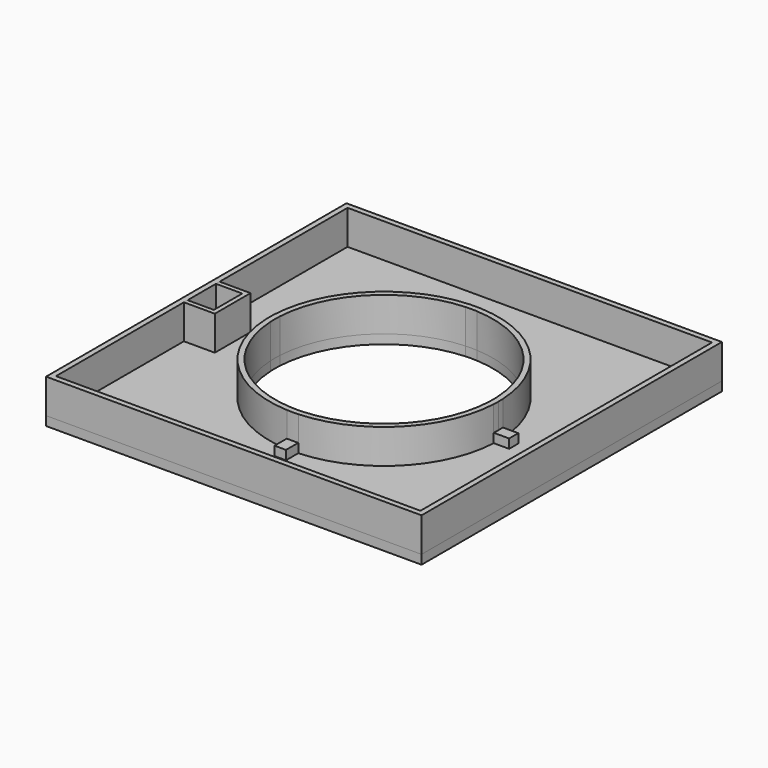
from build123d import *

# Parameters (mm, degrees)
F1_DEPTH = 7.5
F0_W     = 82
F0_H     = 82
F0_R     = 32.8
F0_W_2   = 6.75
F0_H_2   = 9.75
F2_DEPTH = 2
F3_DEPTH = 2
F4_DEPTH = 7.5
F5_T     = -1


# Not quite as in the source:
# - a feature names something its author has since deleted; it is built from what else it names


with BuildPart() as f1:
    # F0 (on Top) → F1 (new body)
    with BuildSketch(Plane.XY):
        with BuildLine():
            ThreePointArc((-24.9687304443, -1.25), (-17.6776695297, -17.6776695297), (-1.25, -24.9687304443))
            Line((-1.25, -24.9687304443), (-1.25, -23.7671517015))
            ThreePointArc((-1.25, -23.7671517015), (-16.8291413922, -16.8291413922), (-23.7671517015, -1.25))
            Line((-23.7671517015, -1.25), (-24.9687304443, -1.25))
        make_face()
        with BuildLine():
            Line((-1.25, 23.7671517015), (-1.25, 24.9687304443))
            ThreePointArc((-1.25, 24.9687304443), (-17.6776695297, 17.6776695297), (-24.9687304443, 1.25))
            Line((-24.9687304443, 1.25), (-23.7671517015, 1.25))
            ThreePointArc((-23.7671517015, 1.25), (-16.8291413922, 16.8291413922), (-1.25, 23.7671517015))
        make_face()
        with BuildLine():
            Line((23.7671517015, 1.25), (24.9687304443, 1.25))
            ThreePointArc((24.9687304443, 1.25), (17.6776695297, 17.6776695297), (1.25, 24.9687304443))
            Line((1.25, 24.9687304443), (1.25, 23.7671517015))
            ThreePointArc((1.25, 23.7671517015), (16.8291413922, 16.8291413922), (23.7671517015, 1.25))
        make_face()
        with BuildLine():
            ThreePointArc((1.25, -24.9687304443), (17.6776695297, -17.6776695297), (24.9687304443, -1.25))
            Line((24.9687304443, -1.25), (23.7671517015, -1.25))
            ThreePointArc((23.7671517015, -1.25), (16.8291413922, -16.8291413922), (1.25, -23.7671517015))
            Line((1.25, -23.7671517015), (1.25, -24.9687304443))
        make_face()
        with BuildLine():
            Line((1.25, 23.7671517015), (1.25, 24.9687304443))
            ThreePointArc((1.25, 24.9687304443), (0, 25), (-1.25, 24.9687304443))
            Line((-1.25, 24.9687304443), (-1.25, 23.7671517015))
            ThreePointArc((-1.25, 23.7671517015), (0, 23.8), (1.25, 23.7671517015))
        make_face()
        with BuildLine():
            ThreePointArc((-1.25, -24.9687304443), (0, -25), (1.25, -24.9687304443))
            Line((1.25, -24.9687304443), (1.25, -23.7671517015))
            ThreePointArc((1.25, -23.7671517015), (0, -23.8), (-1.25, -23.7671517015))
            Line((-1.25, -23.7671517015), (-1.25, -24.9687304443))
        make_face()
        with BuildLine():
            ThreePointArc((24.9687304443, -1.25), (24.9921813885, -0.6251955264), (25, 0))
            ThreePointArc((25, 0), (24.9921813885, 0.6251955264), (24.9687304443, 1.25))
            Line((24.9687304443, 1.25), (23.7671517015, 1.25))
            ThreePointArc((23.7671517015, 1.25), (23.7917865081, 0.6252157649), (23.8, 0))
            ThreePointArc((23.8, 0), (23.7917865081, -0.6252157649), (23.7671517015, -1.25))
            Line((23.7671517015, -1.25), (24.9687304443, -1.25))
        make_face()
        with BuildLine():
            Line((-23.7671517015, 1.25), (-24.9687304443, 1.25))
            ThreePointArc((-24.9687304443, 1.25), (-25, 0), (-24.9687304443, -1.25))
            Line((-24.9687304443, -1.25), (-23.7671517015, -1.25))
            ThreePointArc((-23.7671517015, -1.25), (-23.8, 0), (-23.7671517015, 1.25))
        make_face()
    extrude(amount=F1_DEPTH)


with BuildPart() as f1b:
    # F0 (on Top) → F1, piece 2 (new body)
    with BuildSketch(Plane.XY):
        Rectangle(F0_W, F0_H)
        Polygon((-39.8, 4.875), (-39.8, 39.8), (39.8, 39.8), (39.8, -39.8), (-39.8, -39.8), (-39.8, -4.875), align=None, mode=Mode.SUBTRACT)
    extrude(amount=F1_DEPTH)


with BuildPart() as f2:
    # F0 (on Top) → F2 (new body)
    with BuildSketch(Plane.XY):
        Rectangle(F0_W, F0_H)
        Polygon((-39.8, 4.875), (-39.8, 39.8), (39.8, 39.8), (39.8, -39.8), (-39.8, -39.8), (-39.8, -4.875), align=None, mode=Mode.SUBTRACT)
        Polygon((39.8, 39.8), (-39.8, 39.8), (-39.8, 4.875), (-33.05, 4.875), (-33.05, -4.875), (-39.8, -4.875), (-39.8, -39.8), (39.8, -39.8), align=None)
        Circle(F0_R, mode=Mode.SUBTRACT)
        Circle(F0_R)
        with BuildLine():
            ThreePointArc((1.25, 24.9687304443), (17.6776695297, 17.6776695297), (24.9687304443, 1.25))
            Line((24.9687304443, 1.25), (28.325, 1.25))
            Line((28.325, 1.25), (28.325, -1.25))
            Line((28.325, -1.25), (24.9687304443, -1.25))
            ThreePointArc((24.9687304443, -1.25), (17.6776695297, -17.6776695297), (1.25, -24.9687304443))
            Line((1.25, -24.9687304443), (1.25, -28.325))
            Line((1.25, -28.325), (-1.25, -28.325))
            Line((-1.25, -28.325), (-1.25, -24.9687304443))
            ThreePointArc((-1.25, -24.9687304443), (-17.6776695297, -17.6776695297), (-24.9687304443, -1.25))
            Line((-24.9687304443, -1.25), (-28.325, -1.25))
            Line((-28.325, -1.25), (-28.325, 1.25))
            Line((-28.325, 1.25), (-24.9687304443, 1.25))
            ThreePointArc((-24.9687304443, 1.25), (-17.6776695297, 17.6776695297), (-1.25, 24.9687304443))
            Line((-1.25, 24.9687304443), (-1.25, 28.325))
            Line((-1.25, 28.325), (1.25, 28.325))
            Line((1.25, 28.325), (1.25, 24.9687304443))
        make_face(mode=Mode.SUBTRACT)
        with Locations((-36.425, 0)):
            Rectangle(F0_W_2, F0_H_2)
        with BuildLine():
            Line((23.7671517015, 1.25), (24.9687304443, 1.25))
            ThreePointArc((24.9687304443, 1.25), (17.6776695297, 17.6776695297), (1.25, 24.9687304443))
            Line((1.25, 24.9687304443), (1.25, 23.7671517015))
            ThreePointArc((1.25, 23.7671517015), (16.8291413922, 16.8291413922), (23.7671517015, 1.25))
        make_face()
        with BuildLine():
            Line((-1.25, 23.7671517015), (-1.25, 24.9687304443))
            ThreePointArc((-1.25, 24.9687304443), (-17.6776695297, 17.6776695297), (-24.9687304443, 1.25))
            Line((-24.9687304443, 1.25), (-23.7671517015, 1.25))
            ThreePointArc((-23.7671517015, 1.25), (-16.8291413922, 16.8291413922), (-1.25, 23.7671517015))
        make_face()
        with BuildLine():
            ThreePointArc((-24.9687304443, -1.25), (-17.6776695297, -17.6776695297), (-1.25, -24.9687304443))
            Line((-1.25, -24.9687304443), (-1.25, -23.7671517015))
            ThreePointArc((-1.25, -23.7671517015), (-16.8291413922, -16.8291413922), (-23.7671517015, -1.25))
            Line((-23.7671517015, -1.25), (-24.9687304443, -1.25))
        make_face()
        with BuildLine():
            ThreePointArc((1.25, -24.9687304443), (17.6776695297, -17.6776695297), (24.9687304443, -1.25))
            Line((24.9687304443, -1.25), (23.7671517015, -1.25))
            ThreePointArc((23.7671517015, -1.25), (16.8291413922, -16.8291413922), (1.25, -23.7671517015))
            Line((1.25, -23.7671517015), (1.25, -24.9687304443))
        make_face()
        with BuildLine():
            ThreePointArc((-24.9687304443, -1.25), (-25, 0), (-24.9687304443, 1.25))
            Line((-24.9687304443, 1.25), (-28.325, 1.25))
            Line((-28.325, 1.25), (-28.325, -1.25))
            Line((-28.325, -1.25), (-24.9687304443, -1.25))
        make_face()
        with BuildLine():
            Line((1.25, -28.325), (1.25, -24.9687304443))
            ThreePointArc((1.25, -24.9687304443), (0, -25), (-1.25, -24.9687304443))
            Line((-1.25, -24.9687304443), (-1.25, -28.325))
            Line((-1.25, -28.325), (1.25, -28.325))
        make_face()
        with BuildLine():
            ThreePointArc((-1.25, 24.9687304443), (0, 25), (1.25, 24.9687304443))
            Line((1.25, 24.9687304443), (1.25, 28.325))
            Line((1.25, 28.325), (-1.25, 28.325))
            Line((-1.25, 28.325), (-1.25, 24.9687304443))
        make_face()
        with BuildLine():
            ThreePointArc((24.9687304443, 1.25), (24.9921813885, 0.6251955264), (25, 0))
            ThreePointArc((25, 0), (24.9921813885, -0.6251955264), (24.9687304443, -1.25))
            Line((24.9687304443, -1.25), (28.325, -1.25))
            Line((28.325, -1.25), (28.325, 1.25))
            Line((28.325, 1.25), (24.9687304443, 1.25))
        make_face()
        with BuildLine():
            Line((1.25, 23.7671517015), (1.25, 24.9687304443))
            ThreePointArc((1.25, 24.9687304443), (0, 25), (-1.25, 24.9687304443))
            Line((-1.25, 24.9687304443), (-1.25, 23.7671517015))
            ThreePointArc((-1.25, 23.7671517015), (0, 23.8), (1.25, 23.7671517015))
        make_face()
        with BuildLine():
            Line((-23.7671517015, 1.25), (-24.9687304443, 1.25))
            ThreePointArc((-24.9687304443, 1.25), (-25, 0), (-24.9687304443, -1.25))
            Line((-24.9687304443, -1.25), (-23.7671517015, -1.25))
            ThreePointArc((-23.7671517015, -1.25), (-23.8, 0), (-23.7671517015, 1.25))
        make_face()
        with BuildLine():
            ThreePointArc((-1.25, -24.9687304443), (0, -25), (1.25, -24.9687304443))
            Line((1.25, -24.9687304443), (1.25, -23.7671517015))
            ThreePointArc((1.25, -23.7671517015), (0, -23.8), (-1.25, -23.7671517015))
            Line((-1.25, -23.7671517015), (-1.25, -24.9687304443))
        make_face()
        with BuildLine():
            ThreePointArc((24.9687304443, -1.25), (24.9921813885, -0.6251955264), (25, 0))
            ThreePointArc((25, 0), (24.9921813885, 0.6251955264), (24.9687304443, 1.25))
            Line((24.9687304443, 1.25), (23.7671517015, 1.25))
            ThreePointArc((23.7671517015, 1.25), (23.7917865081, 0.6252157649), (23.8, 0))
            ThreePointArc((23.8, 0), (23.7917865081, -0.6252157649), (23.7671517015, -1.25))
            Line((23.7671517015, -1.25), (24.9687304443, -1.25))
        make_face()
    extrude(amount=-F2_DEPTH)


with BuildPart() as f3:
    # F0 (on Top) → F3 (new body)
    with BuildSketch(Plane.XY):
        with BuildLine():
            ThreePointArc((-24.9687304443, -1.25), (-25, 0), (-24.9687304443, 1.25))
            Line((-24.9687304443, 1.25), (-28.325, 1.25))
            Line((-28.325, 1.25), (-28.325, -1.25))
            Line((-28.325, -1.25), (-24.9687304443, -1.25))
        make_face()
    extrude(amount=F3_DEPTH)


with BuildPart() as f3b:
    # F0 (on Top) → F3, piece 2 (new body)
    with BuildSketch(Plane.XY):
        with BuildLine():
            ThreePointArc((-1.25, 24.9687304443), (0, 25), (1.25, 24.9687304443))
            Line((1.25, 24.9687304443), (1.25, 28.325))
            Line((1.25, 28.325), (-1.25, 28.325))
            Line((-1.25, 28.325), (-1.25, 24.9687304443))
        make_face()
    extrude(amount=F3_DEPTH)


with BuildPart() as f3c:
    # F0 (on Top) → F3, piece 3 (new body)
    with BuildSketch(Plane.XY):
        with BuildLine():
            ThreePointArc((24.9687304443, 1.25), (24.9921813885, 0.6251955264), (25, 0))
            ThreePointArc((25, 0), (24.9921813885, -0.6251955264), (24.9687304443, -1.25))
            Line((24.9687304443, -1.25), (28.325, -1.25))
            Line((28.325, -1.25), (28.325, 1.25))
            Line((28.325, 1.25), (24.9687304443, 1.25))
        make_face()
    extrude(amount=F3_DEPTH)


with BuildPart() as f3d:
    # F0 (on Top) → F3, piece 4 (new body)
    with BuildSketch(Plane.XY):
        with BuildLine():
            Line((1.25, -28.325), (1.25, -24.9687304443))
            ThreePointArc((1.25, -24.9687304443), (0, -25), (-1.25, -24.9687304443))
            Line((-1.25, -24.9687304443), (-1.25, -28.325))
            Line((-1.25, -28.325), (1.25, -28.325))
        make_face()
    extrude(amount=F3_DEPTH)


with BuildPart() as f4:
    # F0 (on Top) → F4 (new body)
    with BuildSketch(Plane.XY):
        with Locations((-36.425, 0)):
            Rectangle(F0_W_2, F0_H_2)
    extrude(amount=F4_DEPTH)

    # F5
    f5_openings = [f4.faces().sort_by_distance(p)[0] for p in [
        (-39.8, 0, 3.75),
        (-36.425, 0, 7.5),
    ]]
    offset(amount=F5_T, openings=f5_openings)


solid = Compound([f1.part, f1b.part, f2.part, f3.part, f3b.part, f3c.part, f3d.part, f4.part])
